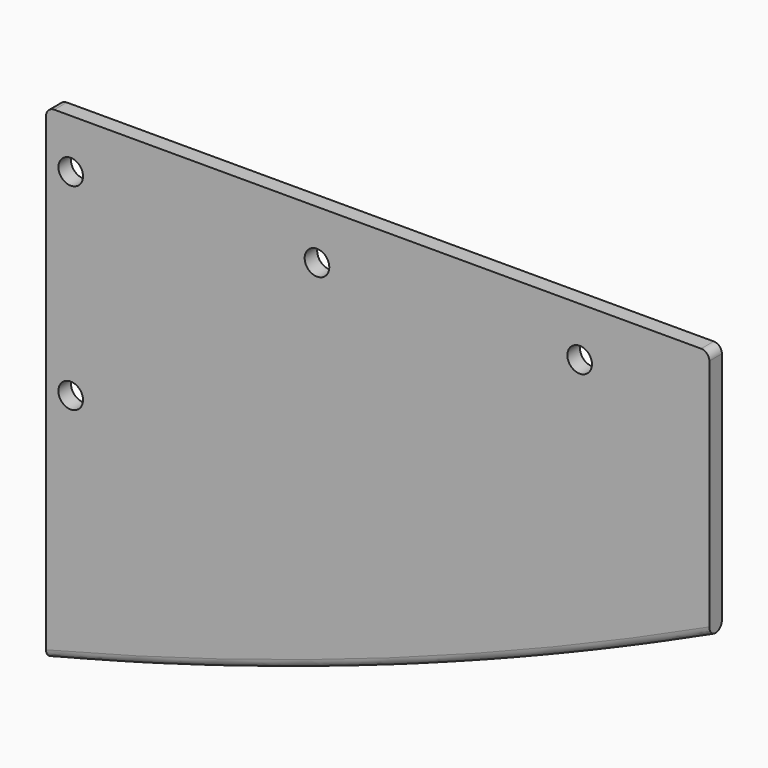
from build123d import *

# Parameters (mm, degrees)
F1_DEPTH = 3.03784
F2_R     = 2.38125
F3_DEPTH = 3.03784
F4_R     = 1.5875
F5_R     = 1.51882


# Not quite as in the source:
# - a fillet or chamfer is up to 0.001 mm smaller than in the source, because OpenCascade refuses the exact size


with BuildPart() as f1:
    # F0 (on Front) → F1 (new body)
    with BuildSketch(Plane.XZ):
        with BuildLine():
            Line((-65.2018, 74.2696), (-65.2018, -19.7612))
            add(Edge.make_bspline(
                [(-65.2018, -19.7612), (-60.7850037253, -18.6171418479), (-51.9575306305, -16.3306106319), (-38.8253253798, -12.61749568), (-25.7966517502, -8.6478861048), (-12.8391741047, -4.4585465011), (0.0137529583, -0.0438991729), (12.7925184797, 4.6371253852), (25.4667360287, 9.5345524455), (38.0928063194, 14.6983578431), (50.6196821862, 20.0682362577), (58.915858645, 23.8585166667), (63.0682, 25.7556)],
                knots=[0, 0, 0, 0, 0.1001945647, 0.2002503103, 0.3002105802, 0.4001552007, 0.5000116128, 0.5999162071, 0.6997672128, 0.7997893994, 0.8997920596, 1, 1, 1, 1], degree=3))
            Line((63.0682, 25.7556), (63.0682, 74.2696))
            Line((63.0682, 74.2696), (-65.2018, 74.2696))
        make_face()
    extrude(amount=F1_DEPTH)

    # F2 (on face) → F3 (cut, through all)
    with BuildSketch(Plane.XZ.offset(3.03784)):
        with Locations((-60.4393, 64.7446)):
            Circle(F2_R)
        with Locations((-60.4393, 26.6446)):
            Circle(F2_R)
        with Locations((-12.8143, 64.7446)):
            Circle(F2_R)
        with Locations((37.9857, 64.7446)):
            Circle(F2_R)
    extrude(amount=-F3_DEPTH, mode=Mode.SUBTRACT)

    # F4
    f4_edges = [f1.edges().sort_by_distance(p)[0] for p in [
        (-65.2018, -1.51892, 74.2696),
        (63.0682, -1.51892, 74.2696),
    ]]
    fillet(f4_edges, radius=F4_R)

    # F5 (radius 1.51892 in the source; OpenCascade refuses exactly that, so slightly less here)
    f5_edges = [f1.edges().sort_by_distance(p)[0] for p in [
        (-0.002981, -3.03784, -0.001058),
        (-0.002981, 0, -0.001058),
    ]]
    fillet(f5_edges, radius=F5_R)


solid = f1.part
